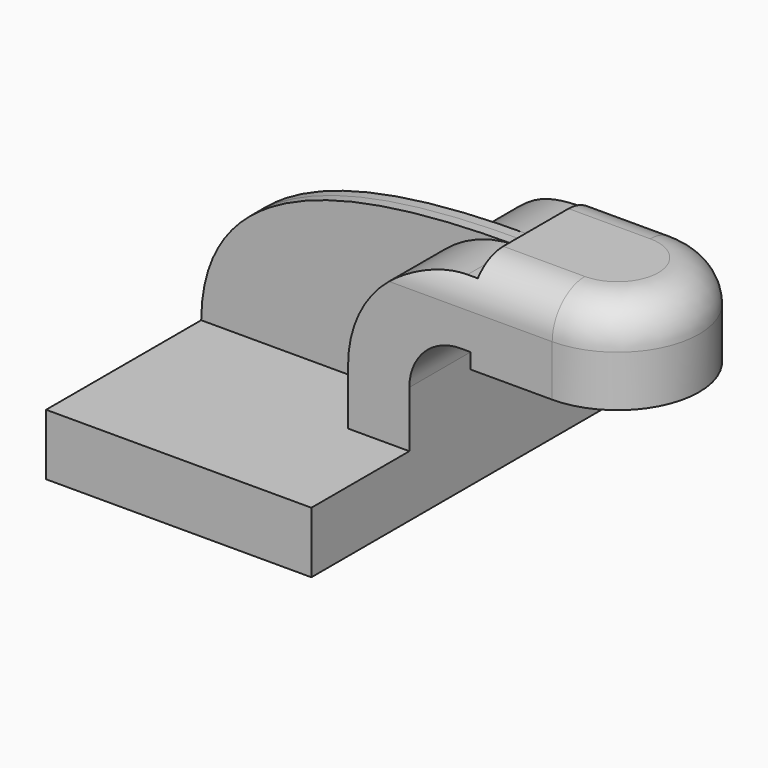
from build123d import *

# Parameters (mm, degrees)
F1_DEPTH = 63.5
F0_W     = 25.4
F0_H     = 4.7752
F0_H_2   = 19.05
F0_H_3   = 4.7498
F2_DEPTH = 25.4
F4_DEPTH = 3.175
F5_R     = 12.7


with BuildPart() as f1:
    # F0 (on Front) → F1 (new body, symmetric)
    with BuildSketch(Plane.XZ):
        Polygon((41.275, -9.525), (41.275, 9.525), (22.225, 9.525), (-41.275, 9.525), (-41.275, -9.525), align=None)
    extrude(amount=F1_DEPTH, both=True)

    # F0 (on Front) → F2 (join, symmetric)
    with BuildSketch(Plane.XZ):
        with BuildLine():
            Line((22.225, 9.525), (41.275, 9.525))
            Line((41.275, 9.525), (41.275, 27.0002))
            ThreePointArc((41.275, 27.0002), (45.9246798487, 38.2255201513), (57.15, 42.8752))
            Line((57.15, 42.8752), (60.325, 42.8752))
            Line((60.325, 42.8752), (60.325, 61.9252))
            Line((60.325, 61.9252), (57.15, 61.9252))
            ThreePointArc((57.15, 61.9252), (32.4542956671, 51.6959043329), (22.225, 27.0002))
            Line((22.225, 27.0002), (22.225, 9.525))
        make_face()
        with Locations((73.025, 40.4876)):
            Rectangle(F0_W, F0_H)
        with Locations((73.025, 52.4002)):
            Rectangle(F0_W, F0_H_2)
        with Locations((73.025, 64.3001)):
            Rectangle(F0_W, F0_H_3)
    extrude(amount=F2_DEPTH, both=True)

    # F0 (on Front) → F3 (revolve)
    with BuildSketch(Plane.XZ):
        Polygon((85.725, 61.9252), (85.725, 42.8752), (85.725, 38.1), (111.125, 38.1), (111.125, 66.675), (85.725, 66.675), align=None)
    revolve(axis=Axis((85.725, 0, 52.3875), (0, 0, 1)))

    # F0 (on Front) → F4 (join, symmetric)
    with BuildSketch(Plane.XZ):
        with BuildLine():
            Line((-41.275, 9.525), (22.225, 9.525))
            Line((22.225, 9.525), (22.225, 27.0002))
            ThreePointArc((22.225, 27.0002), (32.4542956671, 51.6959043329), (57.15, 61.9252))
            add(Edge.make_bspline(
                [(-41.275, 9.525), (-40.8581793308, 53.2651096582), (7.8326556832, 62.0646551251), (57.15, 61.9252)],
                knots=[0, 0, 0, 0, 111.5045361635, 111.5045361635, 111.5045361635, 111.5045361635], degree=3))
        make_face()
    extrude(amount=F4_DEPTH, both=True)

    # F5
    f5_edges = [f1.edges().sort_by_distance(p)[0] for p in [
        (85.725, 25.4, 52.3875),
        (73.025, 25.4, 66.675),
        (73.025, -25.4, 66.675),
        (111.125, 0, 66.675),
    ]]
    fillet(f5_edges, radius=F5_R)


solid = f1.part
